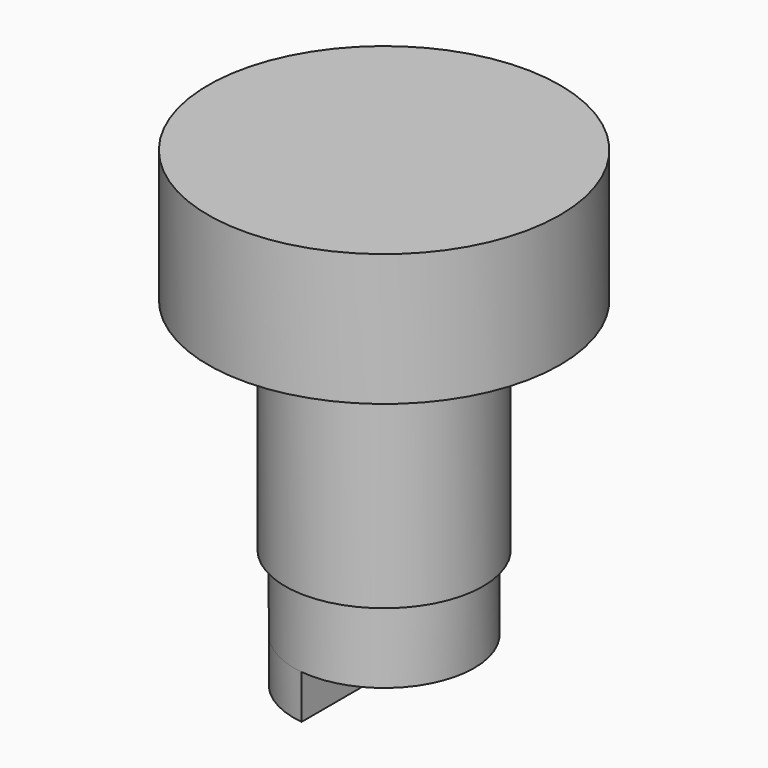
from build123d import *

# Parameters (mm, degrees)
F0_R     = 4.5
F1_DEPTH = 8
F2_R     = 4.5
F3_DEPTH = 2
F4_R     = 8
F5_DEPTH = 6
F6_R     = 4.1
F7_DEPTH = 3.4
F9_DEPTH = 2


# Not quite as in the source:
# - a feature names something its author has since deleted; it is built from what else it names


with BuildPart() as f1:
    # F0 (on Top) → F1 (new body)
    with BuildSketch(Plane.XY):
        Circle(F0_R)
    extrude(amount=F1_DEPTH)

    # F2 (on face) → F3 (join)
    with BuildSketch(Plane.XY.offset(8)):
        Circle(F2_R)
    extrude(amount=F3_DEPTH)

    # F4 (on face) → F5 (join)
    with BuildSketch(Plane.XY.offset(10)):
        Circle(F4_R)
    extrude(amount=F5_DEPTH)

    # F6 (on face) → F7 (join)
    with BuildSketch(Plane(origin=(0, 0, 0), x_dir=(1, 0, 0), z_dir=(0, 0, -1))):
        Circle(F6_R)
    extrude(amount=F7_DEPTH)

    # F8 (on face) → F9 (join)
    with BuildSketch(Plane(origin=(0, 0, -3.4), x_dir=(1, 0, 0), z_dir=(0, 0, -1))):
        with BuildLine():
            Line((-0.499664308, 0), (-0.499664308, 4.0694392217))
            ThreePointArc((-0.499664308, 4.0694392217), (-4.1, 0), (-0.499664308, -4.0694392217))
            Line((-0.499664308, -4.0694392217), (-0.499664308, 0))
        make_face()
    extrude(amount=F9_DEPTH)


solid = f1.part
